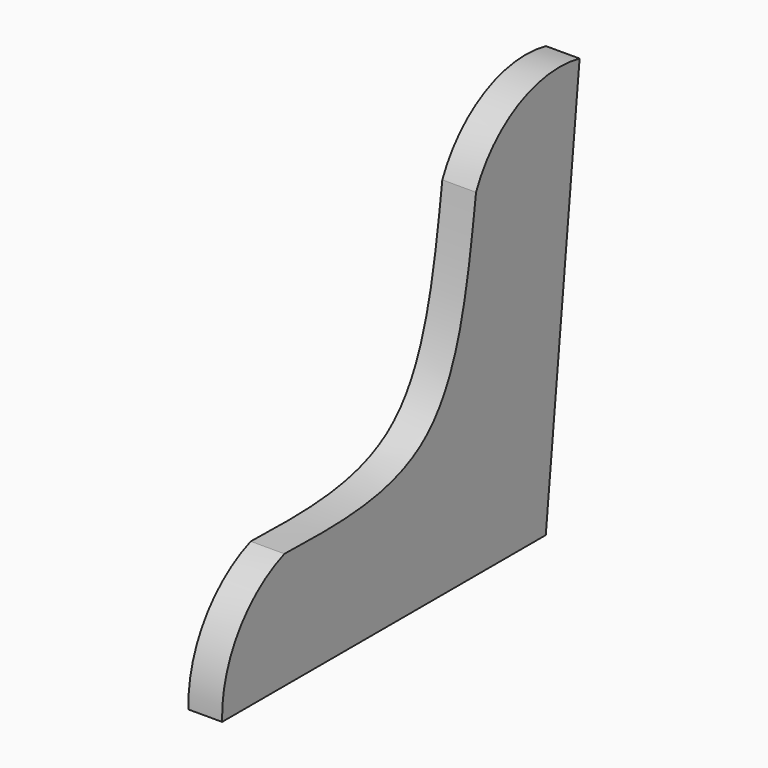
from build123d import *

# Parameters (mm, degrees)
F1_DEPTH = 25.4


with BuildPart() as f1:
    # F0 (on Right) → F1 (new body)
    with BuildSketch(Plane.YZ):
        with BuildLine():
            Line((-304.8, 0), (0, 0))
            Line((0, 0), (31.860275604, 303.1302737082))
            ThreePointArc((31.860275604, 303.1302737082), (-25.6710248369, 296.0445279913), (-65.6702667475, 254.0907561779))
            add(Edge.make_bspline(
                [(-246.146813035, 87.6441970468), (-194.5365692681, 86.4305306387), (-88.5158652272, 83.9373479358), (-73.4183843518, 196.3829828835), (-65.6702667475, 254.0907561779)],
                knots=[0, 0, 0, 0, 0.486794011, 1, 1, 1, 1], degree=3))
            ThreePointArc((-246.146813035, 87.6441970468), (-289.5827369697, 53.2643345738), (-304.8, 0))
        make_face()
    extrude(amount=F1_DEPTH)


solid = f1.part
